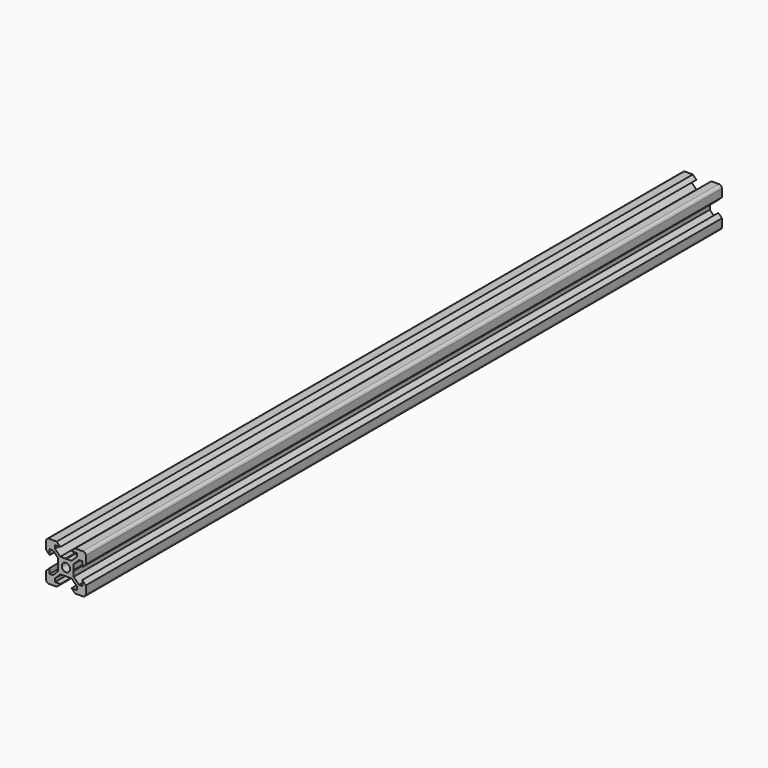
from build123d import *

# Parameters (mm, degrees)
F0_R     = 2.1
F1_DEPTH = 200


# Not quite as in the source:
# - ends of sketch curves that miss each other by under 0.0002 mm in the source are joined


with BuildPart() as f1:
    # F0 (on Front) → F1 (new body, symmetric)
    with BuildSketch(Plane.XZ):
        with BuildLine():
            Line((-4.64, 10.000002), (-8.500001, 10.000002))
            ThreePointArc((-8.500001, 10.000002), (-9.5606615253, 9.5606618182), (-10.000001, 8.500001))
            Line((-10.000001, 8.500001), (-10.000001, 4.640001))
            Line((-10.000001, 4.640001), (-8.199999, 2.840001))
            Line((-8.199999, 2.840001), (-8.199999, 5.499339))
            Line((-8.199999, 5.499339), (-6.56, 5.499339))
            Line((-6.56, 5.499339), (-3.90066, 2.840001))
            Line((-3.90066, 2.840001), (-3.90066, 0.2))
            Line((-3.90066, 0.2), (-3.70066, 0))
            Line((-3.70066, 0), (-3.90066, -0.2))
            Line((-3.90066, -0.2), (-3.90066, -2.840001))
            Line((-3.90066, -2.840001), (-6.56, -5.499341))
            Line((-6.56, -5.499341), (-8.199999, -5.499341))
            Line((-8.199999, -5.499341), (-8.199999, -2.840001))
            Line((-8.199999, -2.840001), (-10.000001, -4.640001))
            Line((-10.000001, -4.640001), (-10.000001, -8.500001))
            ThreePointArc((-10.000001, -8.500001), (-9.5606608182, -9.5606615253), (-8.500001, -10.000001))
            Line((-8.500001, -10.000001), (-4.64, -10.000001))
            Line((-4.64, -10.000001), (-2.84, -8.2))
            Line((-2.84, -8.2), (-5.49934, -8.2))
            Line((-5.49934, -8.2), (-5.49934, -6.560001))
            Line((-5.49934, -6.560001), (-2.84, -3.900661))
            Line((-2.84, -3.900661), (-0.199999, -3.900661))
            Line((-0.199999, -3.900661), (1e-06, -3.700661))
            Line((1e-06, -3.700661), (0.200001, -3.900661))
            Line((0.200001, -3.900661), (2.84, -3.900661))
            Line((2.84, -3.900661), (5.499342, -6.560001))
            Line((5.499342, -6.560001), (5.499342, -8.2))
            Line((5.499342, -8.2), (2.84, -8.2))
            Line((2.84, -8.2), (4.64, -10.000001))
            Line((4.64, -10.000001), (8.500001, -10.000001))
            ThreePointArc((8.500001, -10.000001), (9.5606611718, -9.5606611718), (10.000001, -8.500001))
            Line((10.000001, -8.500001), (10.000001, -4.640001))
            Line((10.000001, -4.640001), (8.200001, -2.840001))
            Line((8.200001, -2.840001), (8.200001, -5.499341))
            Line((8.200001, -5.499341), (6.560002, -5.499341))
            Line((6.560002, -5.499341), (3.90066, -2.840001))
            Line((3.90066, -2.840001), (3.90066, -0.2))
            Line((3.90066, -0.2), (3.70066, 0))
            Line((3.70066, 0), (3.90066, 0.2))
            Line((3.90066, 0.2), (3.90066, 2.840001))
            Line((3.90066, 2.840001), (6.560002, 5.499339))
            Line((6.560002, 5.499339), (8.200001, 5.499339))
            Line((8.200001, 5.499339), (8.200001, 2.840001))
            Line((8.200001, 2.840001), (10.000001, 4.640001))
            Line((10.000001, 4.640001), (10.000001, 8.500002))
            ThreePointArc((10.000001, 8.500002), (9.5606611718, 9.5606621718), (8.500001, 10.000002))
            Line((8.500001, 10.000002), (4.64, 10.000002))
            Line((4.64, 10.000002), (2.84, 8.200002))
            Line((2.84, 8.200002), (5.499342, 8.200002))
            Line((5.499342, 8.200002), (5.499342, 6.559999))
            Line((5.499342, 6.559999), (2.84, 3.900661))
            Line((2.84, 3.900661), (0.200001, 3.900661))
            Line((0.200001, 3.900661), (1e-06, 3.700661))
            Line((1e-06, 3.700661), (-0.199999, 3.900661))
            Line((-0.199999, 3.900661), (-2.84, 3.900661))
            Line((-2.84, 3.900661), (-5.49934, 6.559999))
            Line((-5.49934, 6.559999), (-5.49934, 8.200002))
            Line((-5.49934, 8.200002), (-2.84, 8.200002))
            Line((-2.84, 8.200002), (-4.64, 10.000002))
        make_face()
        with Locations((1e-06, 0)):
            Circle(F0_R, mode=Mode.SUBTRACT)
    extrude(amount=F1_DEPTH, both=True)


solid = f1.part
